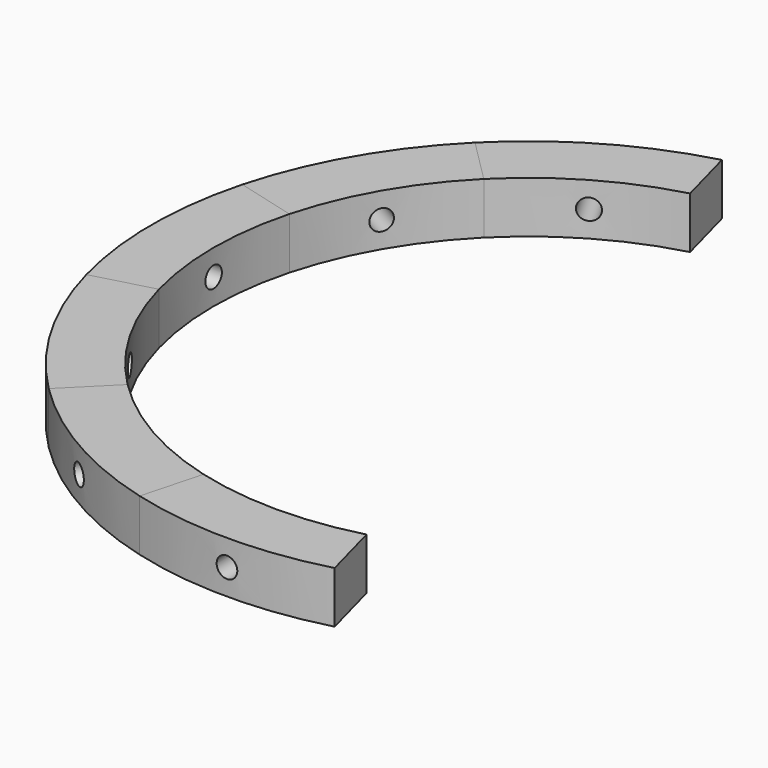
from build123d import *
from build123d import SkipClean  # not in build123d's __all__

# Parameters (mm, degrees)
F1_DEPTH = 15.875
F4_D     = 6.35
F4_DEPTH = 63.246
F4_TIP   = 1.9077324654
F5_COUNT = 6
F5_ANGLE = 150


with BuildPart() as f1:
    # F0 (on Top) → F1 (new body)
    with BuildSketch(Plane.XY):
        with BuildLine():
            ThreePointArc((25.0633892801, -93.5378422033), (0, -96.8375), (-25.0633892801, -93.5378422033))
            Line((-25.0633892801, -93.5378422033), (-29.9938920893, -111.9387291941))
            ThreePointArc((-29.9938920893, -111.9387291941), (0, -115.8875), (29.9938920893, -111.9387291941))
            Line((29.9938920893, -111.9387291941), (25.0633892801, -93.5378422033))
        make_face()
    extrude(amount=F1_DEPTH)

    # F4
    with Locations(Plane.XZ.offset(115.8875)):
        with Locations((0, 7.9375)):
            Hole(F4_D / 2, depth=F4_DEPTH)
            with Locations((0, 0, -(F4_DEPTH + F4_TIP / 2))):  # 118° drill point
                Cone(0, F4_D / 2, F4_TIP, mode=Mode.SUBTRACT)

    # F5: F1 ×6 about axis
    f5_axis = Axis((0, 0, 0), (0, 0, -1))


with BuildPart() as f1_1:
    add(f1.part, clean=False)
    with SkipClean():  # cleaning this boolean's faces spoils the solid; the shape is the same uncleaned
        for i in range(1, F5_COUNT):
            add(f1.part.rotate(f5_axis, i * F5_ANGLE / (F5_COUNT - 1)), clean=False)


solid = f1_1.part
